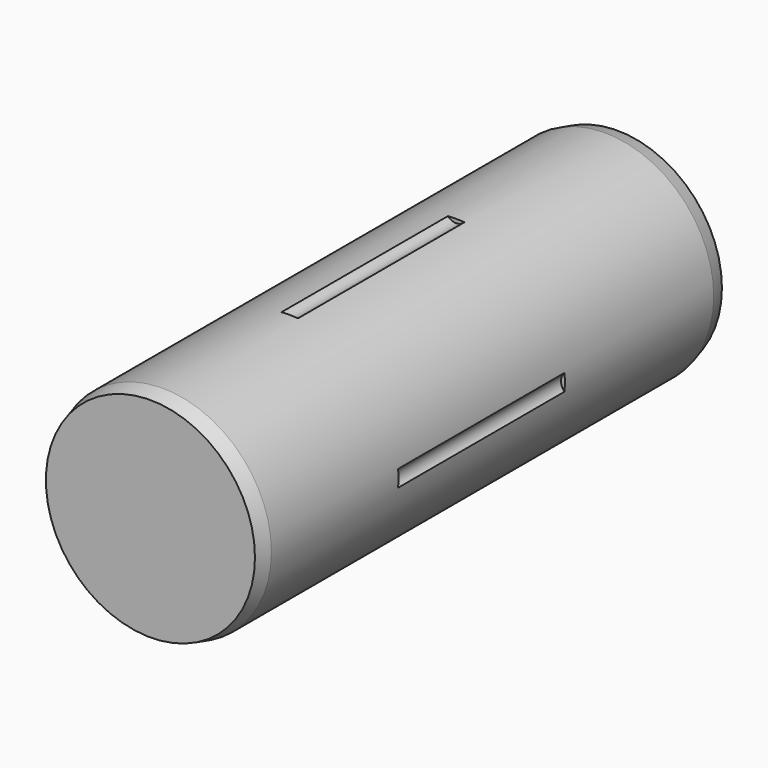
from build123d import *

# Parameters (mm, degrees)
F0_R            = 44.9199
F1_DEPTH        = 241.3
F2_SIZE2        = 1.7014773719
F2_SIZE         = 6.35
F4_R            = 4.7625
F5_DEPTH        = 86
F5_COPIES_COUNT = 4


# Not quite as in the source:
# - a pattern or mirror of a feature is missing from the dataset's text; its kind, count and spacing are read off the source's solid


with BuildPart() as f1:
    # F0 (on Front) → F1 (new body)
    with BuildSketch(Plane.XZ):
        Circle(F0_R)
    extrude(amount=F1_DEPTH)

    # F2
    f2_edges = [f1.edges().sort_by_distance(p)[0] for p in [
        (-44.9199, -241.3, 0),
        (-44.9199, 0, 0),
    ]]
    f2_side = f1.faces().sort_by_distance((-44.9199, -120.65, 0))[0]
    chamfer(f2_edges, length=F2_SIZE, length2=F2_SIZE2, reference=f2_side)

    # F4 (on offset) → F5 (cut)
    with BuildSketch(Plane.XZ.offset(169.3)):
        with Locations((0, -48.0949)):
            Circle(F4_R)
    f5 = extrude(amount=-F5_DEPTH, mode=Mode.SUBTRACT)

    # F5_copies: F5 ×4 about axis
    f5_copies_axis = Axis((0, 0, 0), (0, 1, 0))
    for i in range(1, F5_COPIES_COUNT):
        add(f5.rotate(f5_copies_axis, i * 360 / F5_COPIES_COUNT), mode=Mode.SUBTRACT)


solid = f1.part
